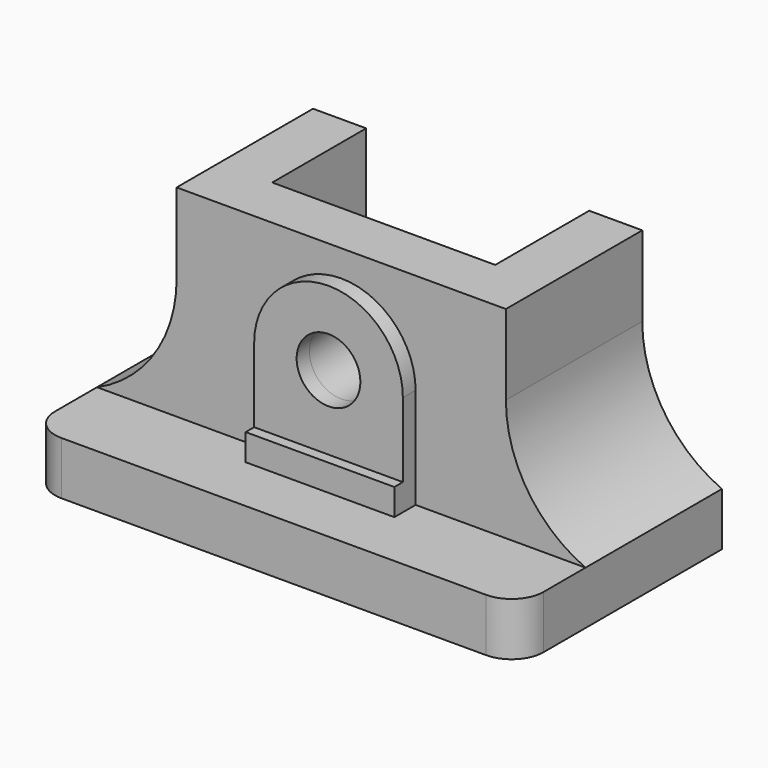
from build123d import *

# Parameters (mm, degrees)
F1_DEPTH    = 48
F2_DEPTH    = 10
F3_T1_DEPTH = 32.1050237641
F4_T1_DEPTH = 32.1050237641
F5_W        = 28
F5_H        = 5
F6_DEPTH    = 5
F5_R        = 6
F7_DEPTH    = 3
F8_DEPTH    = 25


# Not quite as in the source:
# - a fillet or chamfer that OpenCascade refuses, or shapes differently, is made with other operations: its cross-section is extruded or revolved along the edge and cut away or added


with BuildPart() as f1:
    # F0 (on Top) → F1 (new body)
    with BuildSketch(Plane.XY):
        Polygon((31, -8.1050237641), (31, 24), (21, 24), (21, 1.8949762359), (-21, 1.8949762359), (-21, 24), (-31, 24), (-31, -8.1050237641), align=None)
    extrude(amount=F1_DEPTH)

    # F0 (on Top) → F2 (join)
    with BuildSketch(Plane.XY):
        with BuildLine():
            Line((-40, -24), (40, -24))
            ThreePointArc((40, -24), (44.2426406871, -22.2426406871), (46, -18))
            Line((46, -18), (46, 24))
            Line((46, 24), (31, 24))
            Line((31, 24), (31, -8.1050237641))
            Line((31, -8.1050237641), (-31, -8.1050237641))
            Line((-31, -8.1050237641), (-31, 24))
            Line((-31, 24), (-46, 24))
            Line((-46, 24), (-46, -18))
            ThreePointArc((-46, -18), (-44.2426406871, -22.2426406871), (-40, -24))
        make_face()
        Polygon((31, -8.1050237641), (31, 24), (21, 24), (21, 1.8949762359), (-21, 1.8949762359), (-21, 24), (-31, 24), (-31, -8.1050237641), align=None)
    extrude(amount=F2_DEPTH)

    # F3: fillet of radius 25 on 1 edges, made by hand

    # F3_s2 → F3_t1 (join)
    with BuildSketch(Plane.XZ.offset(-24)):
        with BuildLine():
            ThreePointArc((46, 10), (35.0834993366, 19.2198145372), (31, 32.9128784748))
            Line((31, 32.9128784748), (31, 10))
            Line((31, 10), (46, 10))
        make_face()
    extrude(amount=F3_T1_DEPTH)

    # F4: fillet of radius 25 on 1 edges, made by hand

    # F4_s2 → F4_t1 (join)
    with BuildSketch(Plane.XZ.offset(-24)):
        with BuildLine():
            ThreePointArc((-31, 32.9128784748), (-35.0834993366, 19.2198145372), (-46, 10))
            Line((-46, 10), (-31, 10))
            Line((-31, 10), (-31, 32.9128784748))
        make_face()
    extrude(amount=F4_T1_DEPTH)

    # F5 (on face) → F6 (join)
    with BuildSketch(Plane.XZ.offset(8.1050237641)):
        with Locations((0, 12.5)):
            Rectangle(F5_W, F5_H)
    extrude(amount=F6_DEPTH)

    # F5 (on face) → F7 (join)
    with BuildSketch(Plane.XZ.offset(8.1050237641)):
        with BuildLine():
            Line((14, 15), (14, 29))
            ThreePointArc((14, 29), (0, 43), (-14, 29))
            Line((-14, 29), (-14, 15))
            Line((-14, 15), (14, 15))
        make_face()
        with Locations((0, 29)):
            Circle(F5_R, mode=Mode.SUBTRACT)
    extrude(amount=F7_DEPTH)

    # F8 (cut): a face of the model
    f8_faces = [f1.faces().sort_by_distance(p)[0] for p in [
        (0, -8.1050237641, 29),
    ]]
    extrude(f8_faces, amount=-F8_DEPTH, mode=Mode.SUBTRACT)


solid = f1.part
